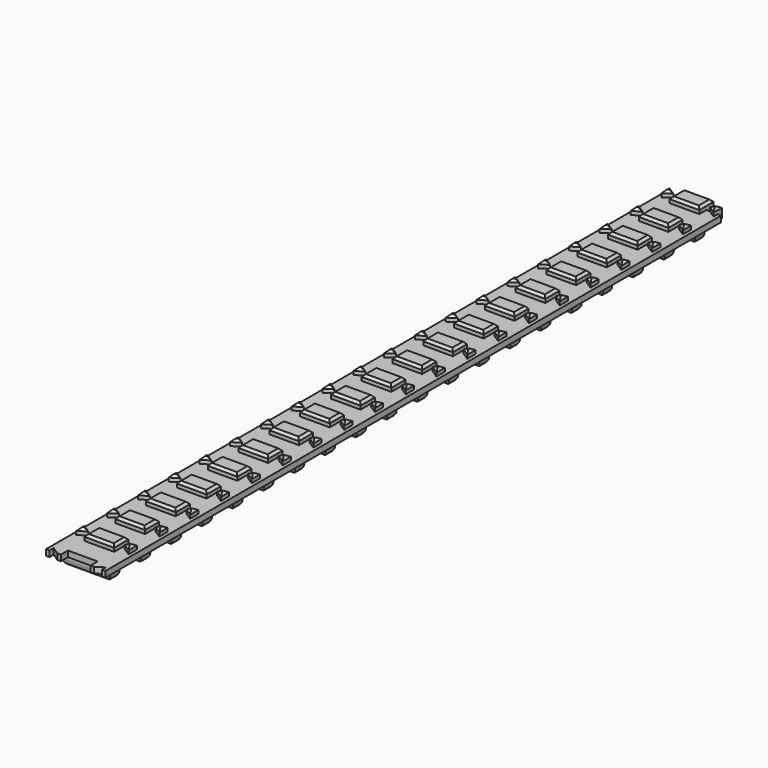
from build123d import *

# Parameters (mm, degrees)
F0_W     = 5
F0_H     = 3
F1_DEPTH = 1
F0_H_2   = 1.5
F2_DEPTH = 2
F3_SIZE  = 0.4
F4_W     = 8
F4_H     = 2
F5_DEPTH = 2
F6_R     = 0.99999


# Not quite as in the source:
# - a fillet or chamfer is up to 0.001 mm smaller than in the source, because OpenCascade refuses the exact size


with BuildPart() as f1:
    # F0 (on Top) → F1 (new body)
    with BuildSketch(Plane.XY):
        Polygon((5, 0), (5, 65), (4.4215835445, 65), (4.4215835445, 64.1277370935), (3.0784164555, 65), (2.5, 65), (2.5, 63.5), (-2.5, 63.5), (-2.5, 65), (-3.0784164555, 65), (-4.4215835445, 64.1277370935), (-4.4215835445, 65), (-5, 65), (-5, -65), (-4.4215835445, -65), (-4.4215835445, -64.1277370935), (-3.0784164555, -65), (-2.5, -65), (-2.5, -63.5), (2.5, -63.5), (2.5, -65), (3.0784164555, -65), (4.4215835445, -64.1277370935), (4.4215835445, -65), (5, -65), align=None)
        Polygon((-4.4215835445, -57.6277370935), (-3.0784164555, -58.5), (-4.4215835445, -59.3722629065), (-4.4215835445, -58.5), align=None, mode=Mode.SUBTRACT)
        Polygon((-4.4215835445, -51.1277370935), (-3.0784164555, -52), (-4.4215835445, -52.8722629065), (-4.4215835445, -52), align=None, mode=Mode.SUBTRACT)
        Polygon((-4.4215835445, -44.6277370935), (-3.0784164555, -45.5), (-4.4215835445, -46.3722629065), (-4.4215835445, -45.5), align=None, mode=Mode.SUBTRACT)
        Polygon((-4.4215835445, -38.1277370935), (-3.0784164555, -39), (-4.4215835445, -39.8722629065), (-4.4215835445, -39), align=None, mode=Mode.SUBTRACT)
        Polygon((-4.4215835445, -31.6277370935), (-3.0784164555, -32.5), (-4.4215835445, -33.3722629065), (-4.4215835445, -32.5), align=None, mode=Mode.SUBTRACT)
        Polygon((-4.4215835445, -25.1277370935), (-3.0784164555, -26), (-4.4215835445, -26.8722629065), (-4.4215835445, -26), align=None, mode=Mode.SUBTRACT)
        Polygon((-4.4215835445, -18.6277370935), (-3.0784164555, -19.5), (-4.4215835445, -20.3722629065), (-4.4215835445, -19.5), align=None, mode=Mode.SUBTRACT)
        Polygon((-4.4215835445, -12.1277370935), (-3.0784164555, -13), (-4.4215835445, -13.8722629065), (-4.4215835445, -13), align=None, mode=Mode.SUBTRACT)
        Polygon((-4.4215835445, -5.6277370935), (-3.0784164555, -6.5), (-4.4215835445, -7.3722629065), (-4.4215835445, -6.5), align=None, mode=Mode.SUBTRACT)
        with Locations((0, -58.5)):
            Rectangle(F0_W, F0_H, mode=Mode.SUBTRACT)
        with Locations((0, -52)):
            Rectangle(F0_W, F0_H, mode=Mode.SUBTRACT)
        with Locations((0, -45.5)):
            Rectangle(F0_W, F0_H, mode=Mode.SUBTRACT)
        with Locations((0, -39)):
            Rectangle(F0_W, F0_H, mode=Mode.SUBTRACT)
        Polygon((4.4215835445, -59.3722629065), (3.0784164555, -58.5), (4.4215835445, -57.6277370935), (4.4215835445, -58.5), align=None, mode=Mode.SUBTRACT)
        Polygon((4.4215835445, -52.8722629065), (3.0784164555, -52), (4.4215835445, -51.1277370935), (4.4215835445, -52), align=None, mode=Mode.SUBTRACT)
        Polygon((4.4215835445, -46.3722629065), (3.0784164555, -45.5), (4.4215835445, -44.6277370935), (4.4215835445, -45.5), align=None, mode=Mode.SUBTRACT)
        Polygon((4.4215835445, -39.8722629065), (3.0784164555, -39), (4.4215835445, -38.1277370935), (4.4215835445, -39), align=None, mode=Mode.SUBTRACT)
        with Locations((0, -32.5)):
            Rectangle(F0_W, F0_H, mode=Mode.SUBTRACT)
        with Locations((0, -26)):
            Rectangle(F0_W, F0_H, mode=Mode.SUBTRACT)
        with Locations((0, -19.5)):
            Rectangle(F0_W, F0_H, mode=Mode.SUBTRACT)
        with Locations((0, -13)):
            Rectangle(F0_W, F0_H, mode=Mode.SUBTRACT)
        with Locations((0, -6.5)):
            Rectangle(F0_W, F0_H, mode=Mode.SUBTRACT)
        Polygon((4.4215835445, -33.3722629065), (3.0784164555, -32.5), (4.4215835445, -31.6277370935), (4.4215835445, -32.5), align=None, mode=Mode.SUBTRACT)
        Polygon((4.4215835445, -26.8722629065), (3.0784164555, -26), (4.4215835445, -25.1277370935), (4.4215835445, -26), align=None, mode=Mode.SUBTRACT)
        Polygon((4.4215835445, -20.3722629065), (3.0784164555, -19.5), (4.4215835445, -18.6277370935), (4.4215835445, -19.5), align=None, mode=Mode.SUBTRACT)
        Polygon((4.4215835445, -13.8722629065), (3.0784164555, -13), (4.4215835445, -12.1277370935), (4.4215835445, -13), align=None, mode=Mode.SUBTRACT)
        Polygon((4.4215835445, -7.3722629065), (3.0784164555, -6.5), (4.4215835445, -5.6277370935), (4.4215835445, -6.5), align=None, mode=Mode.SUBTRACT)
        Polygon((-4.4215835445, 0.8722629065), (-3.0784164555, 0), (-4.4215835445, -0.8722629065), (-4.4215835445, 0), align=None, mode=Mode.SUBTRACT)
        Polygon((-4.4215835445, 6.5), (-4.4215835445, 7.3722629065), (-3.0784164555, 6.5), (-4.4215835445, 5.6277370935), align=None, mode=Mode.SUBTRACT)
        Polygon((-4.4215835445, 13), (-4.4215835445, 13.8722629065), (-3.0784164555, 13), (-4.4215835445, 12.1277370935), align=None, mode=Mode.SUBTRACT)
        Polygon((-4.4215835445, 19.5), (-4.4215835445, 20.3722629065), (-3.0784164555, 19.5), (-4.4215835445, 18.6277370935), align=None, mode=Mode.SUBTRACT)
        Polygon((-4.4215835445, 26), (-4.4215835445, 26.8722629065), (-3.0784164555, 26), (-4.4215835445, 25.1277370935), align=None, mode=Mode.SUBTRACT)
        Polygon((-4.4215835445, 32.5), (-4.4215835445, 33.3722629065), (-3.0784164555, 32.5), (-4.4215835445, 31.6277370935), align=None, mode=Mode.SUBTRACT)
        Polygon((-4.4215835445, 39), (-4.4215835445, 39.8722629065), (-3.0784164555, 39), (-4.4215835445, 38.1277370935), align=None, mode=Mode.SUBTRACT)
        Polygon((-4.4215835445, 45.5), (-4.4215835445, 46.3722629065), (-3.0784164555, 45.5), (-4.4215835445, 44.6277370935), align=None, mode=Mode.SUBTRACT)
        Polygon((-4.4215835445, 52), (-4.4215835445, 52.8722629065), (-3.0784164555, 52), (-4.4215835445, 51.1277370935), align=None, mode=Mode.SUBTRACT)
        Polygon((-4.4215835445, 58.5), (-4.4215835445, 59.3722629065), (-3.0784164555, 58.5), (-4.4215835445, 57.6277370935), align=None, mode=Mode.SUBTRACT)
        Polygon((2.5, 1.5), (2.5, 0), (2.5, -1.5), (-2.5, -1.5), (-2.5, 1.5), align=None, mode=Mode.SUBTRACT)
        with Locations((0, 6.5)):
            Rectangle(F0_W, F0_H, mode=Mode.SUBTRACT)
        with Locations((0, 13)):
            Rectangle(F0_W, F0_H, mode=Mode.SUBTRACT)
        with Locations((0, 19.5)):
            Rectangle(F0_W, F0_H, mode=Mode.SUBTRACT)
        with Locations((0, 26)):
            Rectangle(F0_W, F0_H, mode=Mode.SUBTRACT)
        with Locations((0, 32.5)):
            Rectangle(F0_W, F0_H, mode=Mode.SUBTRACT)
        Polygon((4.4215835445, 0.8722629065), (4.4215835445, 0), (4.4215835445, -0.8722629065), (3.0784164555, 0), align=None, mode=Mode.SUBTRACT)
        Polygon((4.4215835445, 5.6277370935), (3.0784164555, 6.5), (4.4215835445, 7.3722629065), (4.4215835445, 6.5), align=None, mode=Mode.SUBTRACT)
        Polygon((4.4215835445, 12.1277370935), (3.0784164555, 13), (4.4215835445, 13.8722629065), (4.4215835445, 13), align=None, mode=Mode.SUBTRACT)
        Polygon((4.4215835445, 18.6277370935), (3.0784164555, 19.5), (4.4215835445, 20.3722629065), (4.4215835445, 19.5), align=None, mode=Mode.SUBTRACT)
        Polygon((4.4215835445, 25.1277370935), (3.0784164555, 26), (4.4215835445, 26.8722629065), (4.4215835445, 26), align=None, mode=Mode.SUBTRACT)
        Polygon((4.4215835445, 31.6277370935), (3.0784164555, 32.5), (4.4215835445, 33.3722629065), (4.4215835445, 32.5), align=None, mode=Mode.SUBTRACT)
        with Locations((0, 39)):
            Rectangle(F0_W, F0_H, mode=Mode.SUBTRACT)
        with Locations((0, 45.5)):
            Rectangle(F0_W, F0_H, mode=Mode.SUBTRACT)
        with Locations((0, 52)):
            Rectangle(F0_W, F0_H, mode=Mode.SUBTRACT)
        with Locations((0, 58.5)):
            Rectangle(F0_W, F0_H, mode=Mode.SUBTRACT)
        Polygon((4.4215835445, 38.1277370935), (3.0784164555, 39), (4.4215835445, 39.8722629065), (4.4215835445, 39), align=None, mode=Mode.SUBTRACT)
        Polygon((4.4215835445, 44.6277370935), (3.0784164555, 45.5), (4.4215835445, 46.3722629065), (4.4215835445, 45.5), align=None, mode=Mode.SUBTRACT)
        Polygon((4.4215835445, 51.1277370935), (3.0784164555, 52), (4.4215835445, 52.8722629065), (4.4215835445, 52), align=None, mode=Mode.SUBTRACT)
        Polygon((4.4215835445, 57.6277370935), (3.0784164555, 58.5), (4.4215835445, 59.3722629065), (4.4215835445, 58.5), align=None, mode=Mode.SUBTRACT)
    extrude(amount=F1_DEPTH)

    # F0 (on Top) → F2 (join)
    with BuildSketch(Plane.XY):
        Polygon((-4.4215835445, 65), (-3.0784164555, 65), (-4.4215835445, 65.8722629065), align=None)
        Polygon((-4.4215835445, 64.1277370935), (-3.0784164555, 65), (-4.4215835445, 65), align=None)
        with Locations((0, 65.75)):
            Rectangle(F0_W, F0_H_2)
        with Locations((0, 64.25)):
            Rectangle(F0_W, F0_H_2)
        Polygon((3.0784164555, 65), (4.4215835445, 65), (4.4215835445, 65.8722629065), align=None)
        Polygon((4.4215835445, 64.1277370935), (4.4215835445, 65), (3.0784164555, 65), align=None)
        with Locations((0, 58.5)):
            Rectangle(F0_W, F0_H)
        Polygon((4.4215835445, 59.3722629065), (3.0784164555, 58.5), (4.4215835445, 57.6277370935), (4.4215835445, 58.5), align=None)
        Polygon((-3.0784164555, 58.5), (-4.4215835445, 59.3722629065), (-4.4215835445, 58.5), (-4.4215835445, 57.6277370935), align=None)
        Polygon((-3.0784164555, 52), (-4.4215835445, 52.8722629065), (-4.4215835445, 52), (-4.4215835445, 51.1277370935), align=None)
        with Locations((0, 52)):
            Rectangle(F0_W, F0_H)
        Polygon((4.4215835445, 52.8722629065), (3.0784164555, 52), (4.4215835445, 51.1277370935), (4.4215835445, 52), align=None)
        Polygon((-3.0784164555, 45.5), (-4.4215835445, 46.3722629065), (-4.4215835445, 45.5), (-4.4215835445, 44.6277370935), align=None)
        with Locations((0, 45.5)):
            Rectangle(F0_W, F0_H)
        Polygon((4.4215835445, 46.3722629065), (3.0784164555, 45.5), (4.4215835445, 44.6277370935), (4.4215835445, 45.5), align=None)
        Polygon((4.4215835445, 39.8722629065), (3.0784164555, 39), (4.4215835445, 38.1277370935), (4.4215835445, 39), align=None)
        with Locations((0, 39)):
            Rectangle(F0_W, F0_H)
        Polygon((-3.0784164555, 39), (-4.4215835445, 39.8722629065), (-4.4215835445, 39), (-4.4215835445, 38.1277370935), align=None)
        Polygon((-3.0784164555, 32.5), (-4.4215835445, 33.3722629065), (-4.4215835445, 32.5), (-4.4215835445, 31.6277370935), align=None)
        with Locations((0, 32.5)):
            Rectangle(F0_W, F0_H)
        Polygon((4.4215835445, 33.3722629065), (3.0784164555, 32.5), (4.4215835445, 31.6277370935), (4.4215835445, 32.5), align=None)
        with Locations((0, 26)):
            Rectangle(F0_W, F0_H)
        Polygon((-3.0784164555, 26), (-4.4215835445, 26.8722629065), (-4.4215835445, 26), (-4.4215835445, 25.1277370935), align=None)
        Polygon((4.4215835445, 26.8722629065), (3.0784164555, 26), (4.4215835445, 25.1277370935), (4.4215835445, 26), align=None)
        Polygon((-3.0784164555, 19.5), (-4.4215835445, 20.3722629065), (-4.4215835445, 19.5), (-4.4215835445, 18.6277370935), align=None)
        with Locations((0, 19.5)):
            Rectangle(F0_W, F0_H)
        Polygon((4.4215835445, 20.3722629065), (3.0784164555, 19.5), (4.4215835445, 18.6277370935), (4.4215835445, 19.5), align=None)
        with Locations((0, 13)):
            Rectangle(F0_W, F0_H)
        Polygon((-3.0784164555, 13), (-4.4215835445, 13.8722629065), (-4.4215835445, 13), (-4.4215835445, 12.1277370935), align=None)
        Polygon((4.4215835445, 13.8722629065), (3.0784164555, 13), (4.4215835445, 12.1277370935), (4.4215835445, 13), align=None)
        with Locations((0, 6.5)):
            Rectangle(F0_W, F0_H)
        Polygon((-3.0784164555, 6.5), (-4.4215835445, 7.3722629065), (-4.4215835445, 6.5), (-4.4215835445, 5.6277370935), align=None)
        Polygon((4.4215835445, 7.3722629065), (3.0784164555, 6.5), (4.4215835445, 5.6277370935), (4.4215835445, 6.5), align=None)
        Polygon((2.5, -1.5), (2.5, 0), (2.5, 1.5), (-2.5, 1.5), (-2.5, -1.5), align=None)
        Polygon((-4.4215835445, -0.8722629065), (-3.0784164555, 0), (-4.4215835445, 0.8722629065), (-4.4215835445, 0), align=None)
        Polygon((4.4215835445, -0.8722629065), (4.4215835445, 0), (3.0784164555, 0), align=None)
        Polygon((3.0784164555, 0), (4.4215835445, 0), (4.4215835445, 0.8722629065), align=None)
        Polygon((-4.4215835445, -7.3722629065), (-3.0784164555, -6.5), (-4.4215835445, -5.6277370935), (-4.4215835445, -6.5), align=None)
        with Locations((0, -6.5)):
            Rectangle(F0_W, F0_H)
        Polygon((4.4215835445, -5.6277370935), (3.0784164555, -6.5), (4.4215835445, -7.3722629065), (4.4215835445, -6.5), align=None)
        Polygon((4.4215835445, -12.1277370935), (3.0784164555, -13), (4.4215835445, -13.8722629065), (4.4215835445, -13), align=None)
        with Locations((0, -13)):
            Rectangle(F0_W, F0_H)
        Polygon((-4.4215835445, -13.8722629065), (-3.0784164555, -13), (-4.4215835445, -12.1277370935), (-4.4215835445, -13), align=None)
        with Locations((0, -19.5)):
            Rectangle(F0_W, F0_H)
        Polygon((-4.4215835445, -20.3722629065), (-3.0784164555, -19.5), (-4.4215835445, -18.6277370935), (-4.4215835445, -19.5), align=None)
        Polygon((4.4215835445, -18.6277370935), (3.0784164555, -19.5), (4.4215835445, -20.3722629065), (4.4215835445, -19.5), align=None)
        Polygon((4.4215835445, -25.1277370935), (3.0784164555, -26), (4.4215835445, -26.8722629065), (4.4215835445, -26), align=None)
        with Locations((0, -26)):
            Rectangle(F0_W, F0_H)
        Polygon((-4.4215835445, -26.8722629065), (-3.0784164555, -26), (-4.4215835445, -25.1277370935), (-4.4215835445, -26), align=None)
        Polygon((-4.4215835445, -33.3722629065), (-3.0784164555, -32.5), (-4.4215835445, -31.6277370935), (-4.4215835445, -32.5), align=None)
        with Locations((0, -32.5)):
            Rectangle(F0_W, F0_H)
        Polygon((4.4215835445, -31.6277370935), (3.0784164555, -32.5), (4.4215835445, -33.3722629065), (4.4215835445, -32.5), align=None)
        Polygon((-4.4215835445, -39.8722629065), (-3.0784164555, -39), (-4.4215835445, -38.1277370935), (-4.4215835445, -39), align=None)
        with Locations((0, -39)):
            Rectangle(F0_W, F0_H)
        Polygon((4.4215835445, -38.1277370935), (3.0784164555, -39), (4.4215835445, -39.8722629065), (4.4215835445, -39), align=None)
        Polygon((4.4215835445, -44.6277370935), (3.0784164555, -45.5), (4.4215835445, -46.3722629065), (4.4215835445, -45.5), align=None)
        with Locations((0, -45.5)):
            Rectangle(F0_W, F0_H)
        Polygon((-4.4215835445, -46.3722629065), (-3.0784164555, -45.5), (-4.4215835445, -44.6277370935), (-4.4215835445, -45.5), align=None)
        with Locations((0, -52)):
            Rectangle(F0_W, F0_H)
        Polygon((-4.4215835445, -52.8722629065), (-3.0784164555, -52), (-4.4215835445, -51.1277370935), (-4.4215835445, -52), align=None)
        Polygon((4.4215835445, -51.1277370935), (3.0784164555, -52), (4.4215835445, -52.8722629065), (4.4215835445, -52), align=None)
        with Locations((0, -58.5)):
            Rectangle(F0_W, F0_H)
        Polygon((-4.4215835445, -59.3722629065), (-3.0784164555, -58.5), (-4.4215835445, -57.6277370935), (-4.4215835445, -58.5), align=None)
        Polygon((4.4215835445, -57.6277370935), (3.0784164555, -58.5), (4.4215835445, -59.3722629065), (4.4215835445, -58.5), align=None)
    extrude(amount=F2_DEPTH)

    # F3
    f3_edges = [f1.edges().sort_by_distance(p)[0] for p in [
        (0, 66.5, 2),
        (-2.5, 65, 2),
        (0, 63.5, 2),
        (2.5, 65, 2),
        (3.75, 64.563869, 2),
        (3.75, 65.436131, 2),
        (4.421584, 65, 2),
        (-3.75, 65.436131, 2),
        (-4.421584, 65, 2),
        (-3.75, 64.563869, 2),
        (2.5, 58.5, 2),
        (0, 60, 2),
        (-2.5, 58.5, 2),
        (0, 57, 2),
        (-3.75, 58.063869, 2),
        (-3.75, 58.936131, 2),
        (-4.421584, 58.5, 2),
        (4.421584, 58.5, 2),
        (3.75, 58.936131, 2),
        (3.75, 58.063869, 2),
        (4.421584, 52, 2),
        (3.75, 52.436131, 2),
        (3.75, 51.563869, 2),
        (2.5, 52, 2),
        (0, 53.5, 2),
        (-2.5, 52, 2),
        (0, 50.5, 2),
        (-3.75, 51.563869, 2),
        (-3.75, 52.436131, 2),
        (-4.421584, 52, 2),
        (2.5, 45.5, 2),
        (0, 47, 2),
        (-2.5, 45.5, 2),
        (0, 44, 2),
        (2.5, 39, 2),
        (0, 40.5, 2),
        (-2.5, 39, 2),
        (0, 37.5, 2),
        (2.5, 32.5, 2),
        (0, 34, 2),
        (-2.5, 32.5, 2),
        (0, 31, 2),
        (2.5, 26, 2),
        (0, 27.5, 2),
        (-2.5, 26, 2),
        (0, 24.5, 2),
        (2.5, 19.5, 2),
        (0, 21, 2),
        (-2.5, 19.5, 2),
        (0, 18, 2),
        (2.5, 13, 2),
        (0, 14.5, 2),
        (-2.5, 13, 2),
        (0, 11.5, 2),
        (2.5, 6.5, 2),
        (0, 8, 2),
        (-2.5, 6.5, 2),
        (0, 5, 2),
        (2.5, 0, 2),
        (0, 1.5, 2),
        (-2.5, 0, 2),
        (0, -1.5, 2),
        (0, -5, 2),
        (-2.5, -6.5, 2),
        (0, -8, 2),
        (2.5, -6.5, 2),
        (0, -11.5, 2),
        (-2.5, -13, 2),
        (0, -14.5, 2),
        (2.5, -13, 2),
        (0, -18, 2),
        (-2.5, -19.5, 2),
        (0, -21, 2),
        (2.5, -19.5, 2),
        (0, -24.5, 2),
        (-2.5, -26, 2),
        (0, -27.5, 2),
        (2.5, -26, 2),
        (0, -31, 2),
        (-2.5, -32.5, 2),
        (0, -34, 2),
        (2.5, -32.5, 2),
        (0, -37.5, 2),
        (-2.5, -39, 2),
        (0, -40.5, 2),
        (2.5, -39, 2),
        (0, -44, 2),
        (-2.5, -45.5, 2),
        (0, -47, 2),
        (2.5, -45.5, 2),
        (0, -50.5, 2),
        (-2.5, -52, 2),
        (0, -53.5, 2),
        (2.5, -52, 2),
        (0, -57, 2),
        (-2.5, -58.5, 2),
        (0, -60, 2),
        (2.5, -58.5, 2),
        (4.421584, -58.5, 2),
        (3.75, -58.063869, 2),
        (3.75, -58.936131, 2),
        (-3.75, -58.936131, 2),
        (-3.75, -58.063869, 2),
        (-4.421584, -58.5, 2),
        (-3.75, -52.436131, 2),
        (-3.75, -51.563869, 2),
        (-4.421584, -52, 2),
        (4.421584, -52, 2),
        (3.75, -51.563869, 2),
        (3.75, -52.436131, 2),
        (4.421584, -45.5, 2),
        (3.75, -45.063869, 2),
        (3.75, -45.936131, 2),
        (-3.75, -45.936131, 2),
        (-3.75, -45.063869, 2),
        (-4.421584, -45.5, 2),
        (-3.75, -39.436131, 2),
        (-3.75, -38.563869, 2),
        (-4.421584, -39, 2),
        (4.421584, -39, 2),
        (3.75, -38.563869, 2),
        (3.75, -39.436131, 2),
        (4.421584, -32.5, 2),
        (3.75, -32.063869, 2),
        (3.75, -32.936131, 2),
        (-3.75, -32.936131, 2),
        (-3.75, -32.063869, 2),
        (-4.421584, -32.5, 2),
        (3.75, -25.563869, 2),
        (3.75, -26.436131, 2),
        (4.421584, -26, 2),
        (-3.75, -26.436131, 2),
        (-3.75, -25.563869, 2),
        (-4.421584, -26, 2),
        (-3.75, -19.936131, 2),
        (-3.75, -19.063869, 2),
        (-4.421584, -19.5, 2),
        (3.75, -19.063869, 2),
        (3.75, -19.936131, 2),
        (4.421584, -19.5, 2),
        (3.75, -12.563869, 2),
        (3.75, -13.436131, 2),
        (4.421584, -13, 2),
        (-3.75, -13.436131, 2),
        (-3.75, -12.563869, 2),
        (-4.421584, -13, 2),
        (-3.75, -6.936131, 2),
        (-3.75, -6.063869, 2),
        (-4.421584, -6.5, 2),
        (3.75, -6.063869, 2),
        (3.75, -6.936131, 2),
        (4.421584, -6.5, 2),
        (3.75, -0.436131, 2),
        (4.421584, 0, 2),
        (3.75, 0.436131, 2),
        (-4.421584, 0, 2),
        (-3.75, -0.436131, 2),
        (-3.75, 0.436131, 2),
        (-3.75, 6.936131, 2),
        (-4.421584, 6.5, 2),
        (-3.75, 6.063869, 2),
        (3.75, 6.936131, 2),
        (3.75, 6.063869, 2),
        (4.421584, 6.5, 2),
        (3.75, 13.436131, 2),
        (3.75, 12.563869, 2),
        (4.421584, 13, 2),
        (-3.75, 13.436131, 2),
        (-4.421584, 13, 2),
        (-3.75, 12.563869, 2),
        (-3.75, 19.936131, 2),
        (-4.421584, 19.5, 2),
        (-3.75, 19.063869, 2),
        (-3.75, 26.436131, 2),
        (-4.421584, 26, 2),
        (-3.75, 25.563869, 2),
        (3.75, 26.436131, 2),
        (3.75, 25.563869, 2),
        (4.421584, 26, 2),
        (3.75, 19.936131, 2),
        (3.75, 19.063869, 2),
        (4.421584, 19.5, 2),
        (4.421584, 32.5, 2),
        (3.75, 32.936131, 2),
        (3.75, 32.063869, 2),
        (-3.75, 32.063869, 2),
        (-3.75, 32.936131, 2),
        (-4.421584, 32.5, 2),
        (-3.75, 38.563869, 2),
        (-3.75, 39.436131, 2),
        (-4.421584, 39, 2),
        (-3.75, 45.063869, 2),
        (-3.75, 45.936131, 2),
        (-4.421584, 45.5, 2),
        (4.421584, 45.5, 2),
        (3.75, 45.936131, 2),
        (3.75, 45.063869, 2),
        (4.421584, 39, 2),
        (3.75, 39.436131, 2),
        (3.75, 38.563869, 2),
    ]]
    chamfer(f3_edges, length=F3_SIZE)

    # F4 (on face) → F5 (join)
    with BuildSketch(Plane.XY):
        with Locations((0, 61.75)):
            Rectangle(F4_W, F4_H)
        with Locations((0, 55.25)):
            Rectangle(F4_W, F4_H)
        with Locations((0, 48.75)):
            Rectangle(F4_W, F4_H)
        with Locations((0, 42.25)):
            Rectangle(F4_W, F4_H)
        with Locations((0, 35.75)):
            Rectangle(F4_W, F4_H)
        with Locations((0, 29.25)):
            Rectangle(F4_W, F4_H)
        with Locations((0, 22.75)):
            Rectangle(F4_W, F4_H)
        with Locations((0, 16.25)):
            Rectangle(F4_W, F4_H)
        with Locations((0, 9.75)):
            Rectangle(F4_W, F4_H)
        with Locations((0, 3.25)):
            Rectangle(F4_W, F4_H)
        with Locations((0, -3.25)):
            Rectangle(F4_W, F4_H)
        with Locations((0, -9.75)):
            Rectangle(F4_W, F4_H)
        with Locations((0, -16.25)):
            Rectangle(F4_W, F4_H)
        with Locations((0, -22.75)):
            Rectangle(F4_W, F4_H)
        with Locations((0, -29.25)):
            Rectangle(F4_W, F4_H)
        with Locations((0, -35.75)):
            Rectangle(F4_W, F4_H)
        with Locations((0, -42.25)):
            Rectangle(F4_W, F4_H)
        with Locations((0, -48.75)):
            Rectangle(F4_W, F4_H)
        with Locations((0, -55.25)):
            Rectangle(F4_W, F4_H)
        with Locations((0, -61.75)):
            Rectangle(F4_W, F4_H)
    extrude(amount=-F5_DEPTH)

    # F6 (radius 1 in the source; OpenCascade refuses exactly that, so slightly less here)
    f6_edges = [f1.edges().sort_by_distance(p)[0] for p in [
        (-4, 61.75, -2),
        (0, 60.75, -2),
        (4, 61.75, -2),
        (0, 62.75, -2),
        (-4, 55.25, -2),
        (0, 54.25, -2),
        (4, 55.25, -2),
        (0, 56.25, -2),
        (-4, 48.75, -2),
        (0, 47.75, -2),
        (4, 48.75, -2),
        (0, 49.75, -2),
        (-4, 42.25, -2),
        (0, 41.25, -2),
        (4, 42.25, -2),
        (0, 43.25, -2),
        (-4, 35.75, -2),
        (0, 34.75, -2),
        (4, 35.75, -2),
        (0, 36.75, -2),
        (-4, 29.25, -2),
        (0, 28.25, -2),
        (4, 29.25, -2),
        (0, 30.25, -2),
        (-4, 22.75, -2),
        (0, 21.75, -2),
        (4, 22.75, -2),
        (0, 23.75, -2),
        (-4, 16.25, -2),
        (0, 15.25, -2),
        (4, 16.25, -2),
        (0, 17.25, -2),
        (-4, 9.75, -2),
        (0, 8.75, -2),
        (4, 9.75, -2),
        (0, 10.75, -2),
        (-4, 3.25, -2),
        (0, 2.25, -2),
        (4, 3.25, -2),
        (0, 4.25, -2),
        (-4, -3.25, -2),
        (0, -4.25, -2),
        (4, -3.25, -2),
        (0, -2.25, -2),
        (-4, -9.75, -2),
        (0, -10.75, -2),
        (4, -9.75, -2),
        (0, -8.75, -2),
        (-4, -16.25, -2),
        (0, -17.25, -2),
        (4, -16.25, -2),
        (0, -15.25, -2),
        (-4, -22.75, -2),
        (0, -23.75, -2),
        (4, -22.75, -2),
        (0, -21.75, -2),
        (-4, -29.25, -2),
        (0, -30.25, -2),
        (4, -29.25, -2),
        (0, -28.25, -2),
        (-4, -35.75, -2),
        (0, -36.75, -2),
        (4, -35.75, -2),
        (0, -34.75, -2),
        (-4, -42.25, -2),
        (0, -43.25, -2),
        (4, -42.25, -2),
        (0, -41.25, -2),
        (-4, -48.75, -2),
        (0, -49.75, -2),
        (4, -48.75, -2),
        (0, -47.75, -2),
        (-4, -55.25, -2),
        (0, -56.25, -2),
        (4, -55.25, -2),
        (0, -54.25, -2),
        (-4, -61.75, -2),
        (0, -62.75, -2),
        (4, -61.75, -2),
        (0, -60.75, -2),
    ]]
    fillet(f6_edges, radius=F6_R)


solid = f1.part
